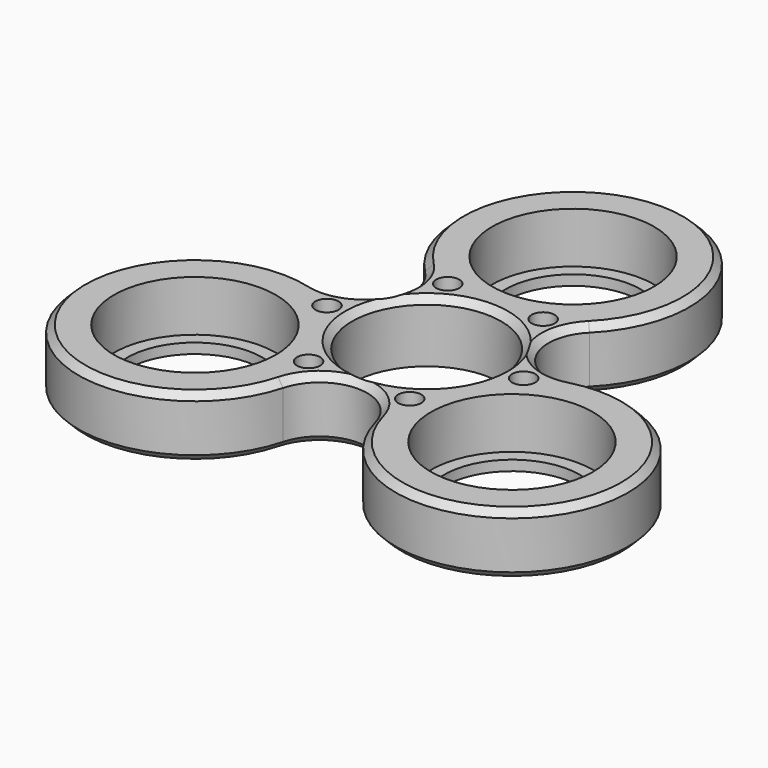
from build123d import *

# Parameters (mm, degrees)
F0_R     = 11.95
F0_R_2   = 1.705642275
F0_R_3   = 11
F1_DEPTH = 9
F2_SIZE  = 1
F0_R_4   = 10
F3_DEPTH = 1.5


# Not quite as in the source:
# - a fillet or chamfer that OpenCascade refuses, or shapes differently, is made with other operations: its cross-section is extruded or revolved along the edge and cut away or added


with BuildPart() as f1:
    # F0 (on Top) → F1 (new body)
    with BuildSketch(Plane.XY):
        with BuildLine():
            ThreePointArc((18.9439392787, 3.0656279209), (11.0053071194, 6.3539170279), (12.1268812973, 14.8731187027))
            ThreePointArc((12.1268812973, 14.8731187027), (0, 44.15), (-12.1268812973, 14.8731187027))
            ThreePointArc((-12.1268812973, 14.8731187027), (-11.0053071194, 6.3539170279), (-18.9439392787, 3.0656279209))
            ThreePointArc((-18.9439392787, 3.0656279209), (-38.2350215771, -22.075), (-6.8170579813, -17.9387466235))
            ThreePointArc((-6.8170579813, -17.9387466235), (0, -12.7078340558), (6.8170579813, -17.9387466235))
            ThreePointArc((6.8170579813, -17.9387466235), (38.2350215771, -22.075), (18.9439392787, 3.0656279209))
        make_face()
        with Locations((-23.3826859022, -13.5)):
            Circle(F0_R, mode=Mode.SUBTRACT)
        with Locations((-7.4659583891, -12.4409667216)):
            Circle(F0_R_2, mode=Mode.SUBTRACT)
        with Locations((-14.5071724231, -0.2452262678)):
            Circle(F0_R_2, mode=Mode.SUBTRACT)
        with Locations((7.4659583891, -12.4409667216)):
            Circle(F0_R_2, mode=Mode.SUBTRACT)
        with Locations((23.3826859022, -13.5)):
            Circle(F0_R, mode=Mode.SUBTRACT)
        Circle(F0_R_3, mode=Mode.SUBTRACT)
        with Locations((14.5071724231, -0.2452262678)):
            Circle(F0_R_2, mode=Mode.SUBTRACT)
        with Locations((-7.041214034, 12.6861929893)):
            Circle(F0_R_2, mode=Mode.SUBTRACT)
        with Locations((7.041214034, 12.6861929893)):
            Circle(F0_R_2, mode=Mode.SUBTRACT)
        with Locations((0, 27)):
            Circle(F0_R, mode=Mode.SUBTRACT)
    extrude(amount=F1_DEPTH)

    # F2
    f2_edges = [f1.edges().sort_by_distance(p)[0] for p in [
        (-38.235022, -22.075, 9),
        (0, -12.707834, 9),
        (38.235022, -22.075, 9),
        (38.235022, -22.075, 0),
        (0, -12.707834, 0),
        (-38.235022, -22.075, 0),
        (-11.005307, 6.353917, 9),
        (-11.005307, 6.353917, 0),
        (0, 44.15, 0),
        (0, 44.15, 9),
        (11.005307, 6.353917, 9),
        (11.005307, 6.353917, 0),
    ]]
    chamfer(f2_edges, length=F2_SIZE)

    # F0 (on Top) → F3 (join)
    with BuildSketch(Plane.XY):
        with Locations((0, 27)):
            Circle(F0_R)
        with Locations((0, 27)):
            Circle(F0_R_4, mode=Mode.SUBTRACT)
        with Locations((-23.3826859022, -13.5)):
            Circle(F0_R)
        with Locations((-23.3826859022, -13.5)):
            Circle(F0_R_4, mode=Mode.SUBTRACT)
        with Locations((23.3826859022, -13.5)):
            Circle(F0_R)
        with Locations((23.3826859022, -13.5)):
            Circle(F0_R_4, mode=Mode.SUBTRACT)
    extrude(amount=F3_DEPTH)

    # F4: chamfer of 1 on 1 edges, made by hand

    # F4_s1 → F4_t2 (revolve, cut)
    with BuildSketch(Plane.XZ):
        Polygon((12, 9), (11, 8), (11, 9), align=None)
    revolve(axis=Axis((0, 0, 9), (0, 0, 1)), mode=Mode.SUBTRACT)


solid = f1.part
